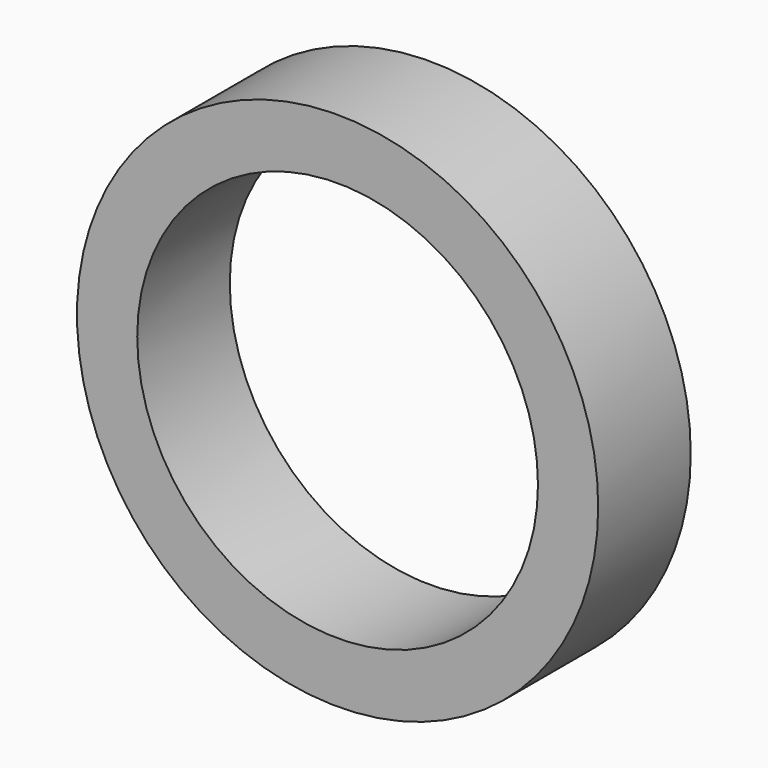
from build123d import *

# Parameters (mm, degrees)
F0_R     = 14.3048091379
F0_R_2   = 10.9982
F3_DEPTH = 6.35


# Not quite as in the source:
# - a feature of the source that left no trace in its solid (it failed there, or was rolled back) is left out


with BuildPart() as f3:
    # F0 (on Front) → F3 (new body)
    with BuildSketch(Plane.XZ):
        Circle(F0_R)
        Circle(F0_R_2, mode=Mode.SUBTRACT)
    extrude(amount=F3_DEPTH)


solid = f3.part
